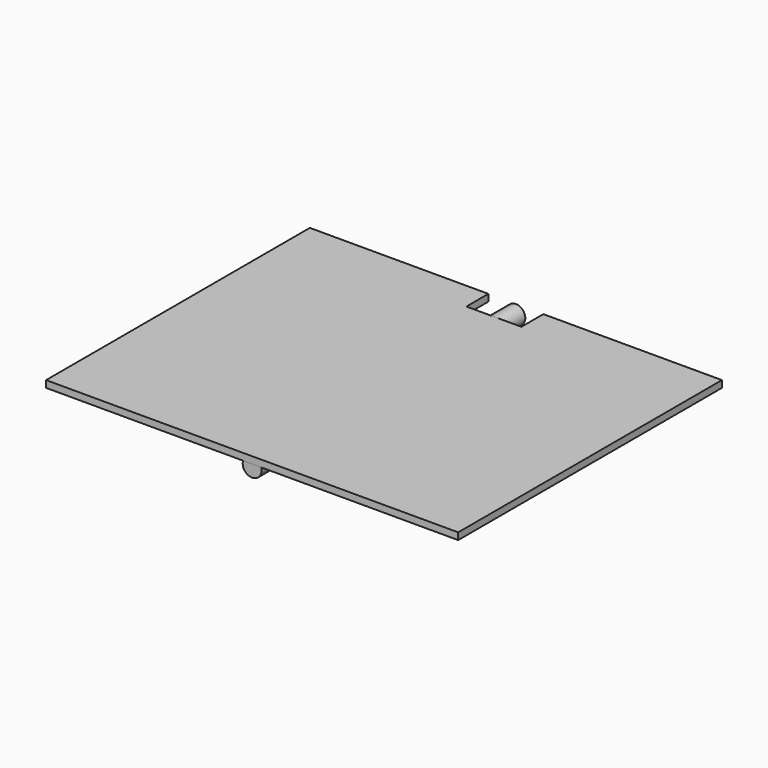
from build123d import *

# Parameters (mm, degrees)
F0_R     = 17.4625
F1_DEPTH = 50.8
F3_DEPTH = 558.8
F4_W     = 762
F4_H     = 12.7
F5_DEPTH = 609.6
F6_W     = 101.6
F6_H     = 50.8
F7_DEPTH = 25.4


with BuildPart() as f1:
    # F0 (on Front) → F1 (new body)
    with BuildSketch(Plane.XZ):
        Circle(F0_R)
    extrude(amount=F1_DEPTH)

    # F2 (on face) → F3 (join)
    with BuildSketch(Plane.XZ.offset(50.8)):
        with BuildLine():
            Line((16.8005208253, 4.7625), (-16.8005208253, 4.7625))
            ThreePointArc((-16.8005208253, 4.7625), (0, -17.4625), (16.8005208253, 4.7625))
        make_face()
    extrude(amount=F3_DEPTH)


with BuildPart() as f5:
    # F4 (on Front) → F5 (new body)
    with BuildSketch(Plane.XZ):
        with Locations((0, 11.1125)):
            Rectangle(F4_W, F4_H)
    extrude(amount=F5_DEPTH)

    # F6 (on face) → F7 (cut)
    with BuildSketch(Plane.XY.offset(17.4625)):
        with Locations((0, -25.4)):
            Rectangle(F6_W, F6_H)
    extrude(amount=-F7_DEPTH, mode=Mode.SUBTRACT)


solid = Compound([f1.part, f5.part])
